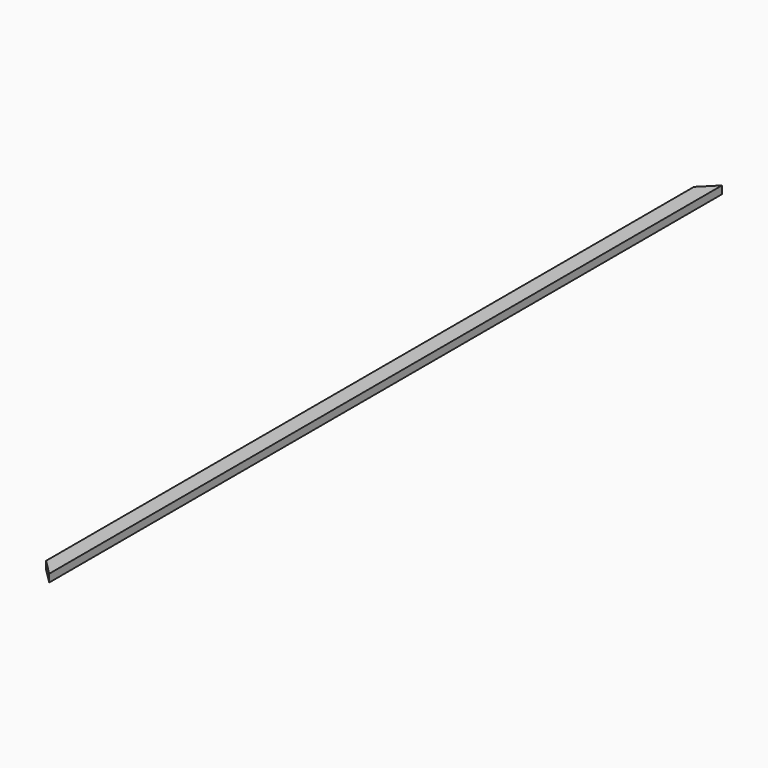
from build123d import *

# Parameters (mm, degrees)
F0_W     = 50.8
F0_H     = 25.4
F1_DEPTH = 2743.2
F2_SIZE  = 50.79999
F3_SIZE  = 50.79999


# Not quite as in the source:
# - a fillet or chamfer is up to 0.001 mm smaller than in the source, because OpenCascade refuses the exact size


with BuildPart() as f1:
    # F0 (on Front) → F1 (new body)
    with BuildSketch(Plane.XZ):
        with Locations((-1.9975652898, 11.9262542576)):
            Rectangle(F0_W, F0_H)
    extrude(amount=F1_DEPTH)

    # F2 (size 50.8 in the source; OpenCascade refuses exactly that, so slightly less here)
    f2_edges = [f1.edges().sort_by_distance(p)[0] for p in [
        (-27.397565, 0, 11.926254),
    ]]
    chamfer(f2_edges, length=F2_SIZE)

    # F3 (size 50.8 in the source; OpenCascade refuses exactly that, so slightly less here)
    f3_edges = [f1.edges().sort_by_distance(p)[0] for p in [
        (-27.397565, -2743.2, 11.926254),
    ]]
    chamfer(f3_edges, length=F3_SIZE)


solid = f1.part
